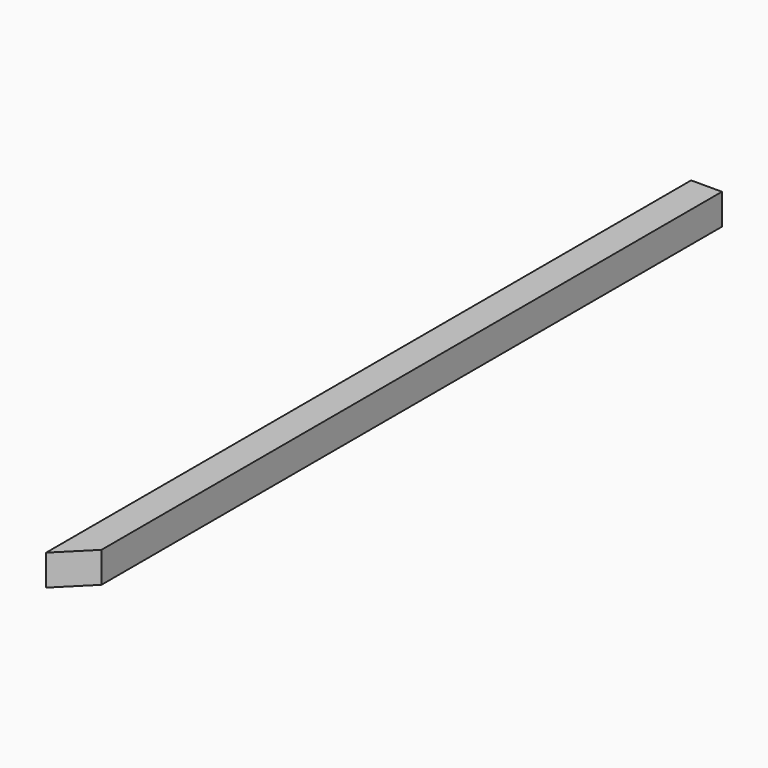
from build123d import *

# Parameters (mm, degrees)
F0_W     = 17.4625
F0_H     = 17.4625
F1_DEPTH = 457.2
F3_DEPTH = 17.4625


# Not quite as in the source:
# - a length typed as a fraction of an inch, garbled in the dataset ("3 / 203.2 mm" for 3/8 in), is restored


with BuildPart() as f1:
    # F0 (on Front) → F1 (new body)
    with BuildSketch(Plane.XZ):
        Rectangle(F0_W, F0_H)
    extrude(amount=F1_DEPTH)

    # F2 (on face) → F3 (cut)
    with BuildSketch(Plane(origin=(0, 0, -8.73125), x_dir=(1, 0, 0), z_dir=(0, 0, -1))):
        Polygon((8.73125, 457.2), (-8.73125, 457.2), (8.73125, 439.7375), align=None)
    extrude(amount=-F3_DEPTH, mode=Mode.SUBTRACT)


solid = f1.part
